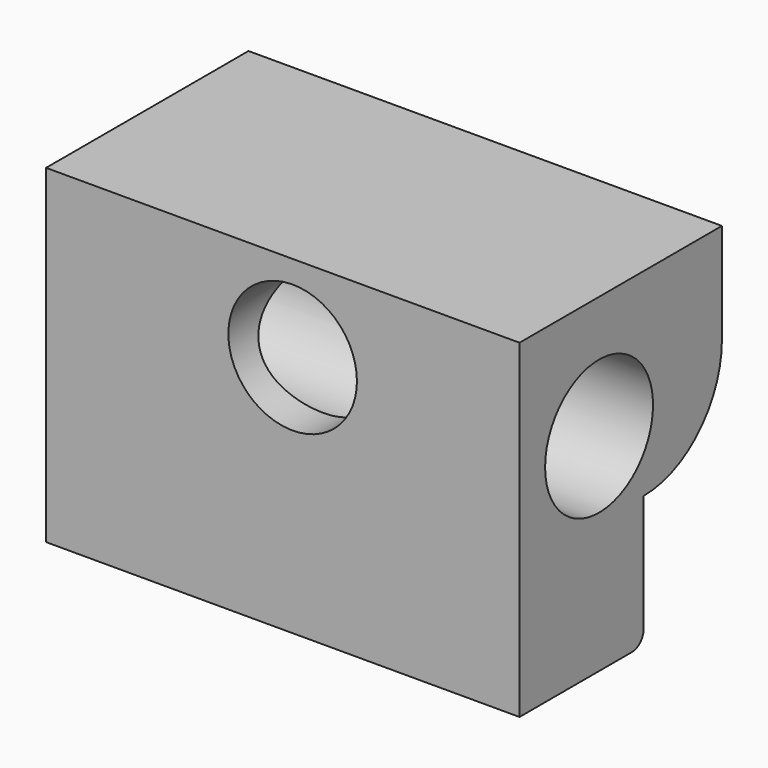
from build123d import *

# Parameters (mm, degrees)
F0_W        = 1544.7841286659
F0_H        = 645.8633244038
F0_R        = 209.7838577095
F1_DEPTH    = 825.5
F2_T1_DEPTH = 3139.1307652571
F3_DEPTH    = 429.26
F4_R        = 220.0590869867
F5_DEPTH    = 1765.3
F6_R        = 48.26
F4_R_2      = 121.9408524026
F7_DEPTH    = 599.44


# Not quite as in the source:
# - a fillet or chamfer that OpenCascade refuses, or shapes differently, is made with other operations: its cross-section is extruded or revolved along the edge and cut away or added


with BuildPart() as f1:
    # F0 (on Front) → F1 (new body)
    with BuildSketch(Plane.XZ):
        with Locations((-71.7625916004, 26.4388471842)):
            Rectangle(F0_W, F0_H)
        with Locations((-39.6583005786, 66.097125411)):
            Circle(F0_R, mode=Mode.SUBTRACT)
    extrude(amount=F1_DEPTH)

    # F2: fillet of radius 318.8693273182 on 1 edges, made by hand

    # F2_s2 → F2_t1 (cut)
    with BuildSketch(Plane.YZ.offset(-1641.327974229)):
        with BuildLine():
            ThreePointArc((-318.8693273182, -296.4928150177), (-93.3946636591, -203.0981513586), (0, 22.3765123005))
            Line((0, 22.3765123005), (0, -296.4928150177))
            Line((0, -296.4928150177), (-318.8693273182, -296.4928150177))
        make_face()
    extrude(amount=F2_T1_DEPTH, mode=Mode.SUBTRACT)

    # F3 (add): a face of the model
    f3_faces = [f1.faces().sort_by_distance(p)[0] for p in [
        (-71.7625916004, -572.1846636591, -296.4928150177),
    ]]
    extrude(f3_faces, amount=F3_DEPTH)

    # F4 (on face) → F5 (cut)
    with BuildSketch(Plane(origin=(-844.1546559334, 0, 0), x_dir=(0, -1, 0), z_dir=(-1, 0, 0))):
        with Locations((501.0944604874, -50.760243088)):
            Circle(F4_R)
    extrude(amount=-F5_DEPTH, mode=Mode.SUBTRACT)

    # F6
    f6_edges = [f1.edges().sort_by_distance(p)[0] for p in [
        (-71.762592, -318.869327, -725.752815),
    ]]
    fillet(f6_edges, radius=F6_R)

    # F4 (on face) → F7 (cut)
    with BuildSketch(Plane(origin=(-844.1546559334, 0, 0), x_dir=(0, -1, 0), z_dir=(-1, 0, 0))):
        with Locations((561.931848526, -504.8967003822)):
            Circle(F4_R_2)
    extrude(amount=-F7_DEPTH, mode=Mode.SUBTRACT)


solid = f1.part
